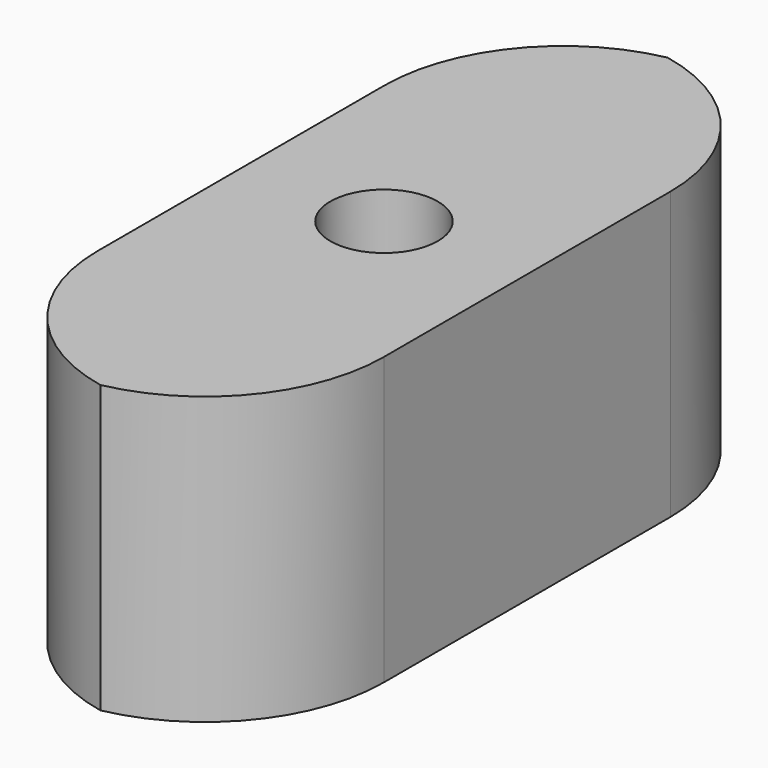
from build123d import *

# Parameters (mm, degrees)
F0_W        = 8
F0_H        = 20
F1_DEPTH    = 8
F2_T1_DEPTH = 33
F3_R        = 1.5
F4_DEPTH    = 7
F5_R        = 2
F5_R_2      = 1.5
F6_DEPTH    = 3


# Not quite as in the source:
# - a fillet or chamfer that OpenCascade refuses, or shapes differently, is made with other operations: its cross-section is extruded or revolved along the edge and cut away or added


with BuildPart() as f1:
    # F0 (on Top) → F1 (new body)
    with BuildSketch(Plane.XY):
        Rectangle(F0_W, F0_H)
    extrude(amount=F1_DEPTH)

    # F2: fillet of radius 5 on 4 edges, made by hand

    # F2_s2 → F2_t1 (cut)
    with BuildSketch(Plane.XY.offset(-12.5)):
        with BuildLine():
            ThreePointArc((4, -5), (2.5355339059, -8.5355339059), (-1, -10))
            Line((-1, -10), (4, -10))
            Line((4, -10), (4, -5))
        make_face()
        with BuildLine():
            ThreePointArc((-4, -5), (-2.5355339059, -8.5355339059), (1, -10))
            Line((1, -10), (-4, -10))
            Line((-4, -10), (-4, -5))
        make_face()
        with BuildLine():
            ThreePointArc((4, 5), (2.5355339059, 8.5355339059), (-1, 10))
            Line((-1, 10), (4, 10))
            Line((4, 10), (4, 5))
        make_face()
        with BuildLine():
            ThreePointArc((1, 10), (-2.5355339059, 8.5355339059), (-4, 5))
            Line((-4, 5), (-4, 10))
            Line((-4, 10), (1, 10))
        make_face()
    extrude(amount=F2_T1_DEPTH, mode=Mode.SUBTRACT)

    # F3 (on face) → F4 (cut)
    with BuildSketch(Plane.XY.offset(8)):
        Circle(F3_R)
    extrude(amount=-F4_DEPTH, mode=Mode.SUBTRACT)

    # F5 (on face) → F6 (cut)
    with BuildSketch(Plane.XY.offset(1)):
        Circle(F5_R)
        Circle(F5_R_2, mode=Mode.SUBTRACT)
    extrude(amount=F6_DEPTH, mode=Mode.SUBTRACT)


solid = f1.part
